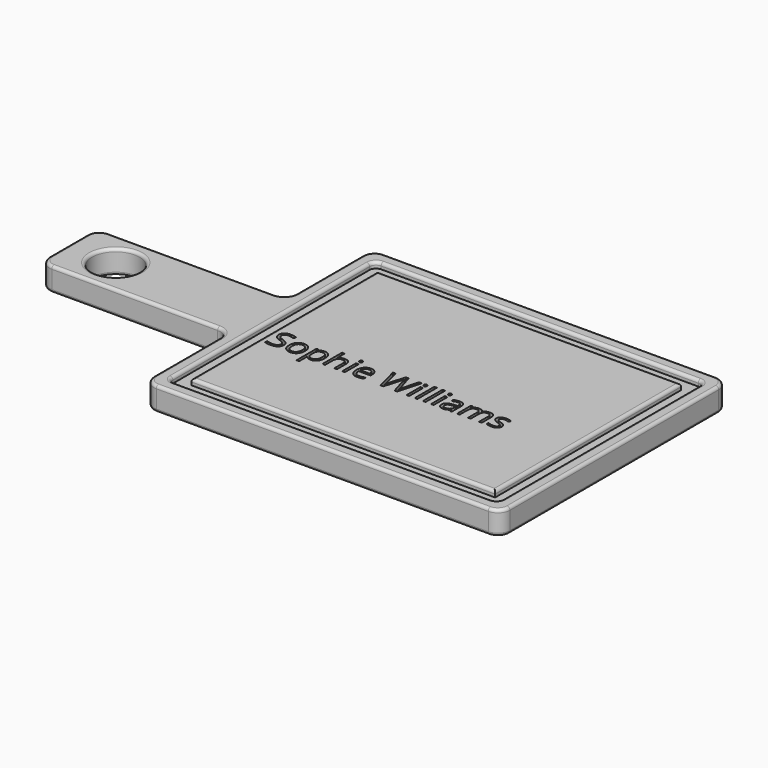
from build123d import *

# Parameters (mm, degrees)
F1_DEPTH      = 25.4
F2_R          = 25.4
F3_DEPTH      = 25.4
F5_DEPTH      = 6.35
F6_R          = 6.8679547422
F7_R          = 12.8774151417
F8_R          = 3.175
F9_TEXT_SIZE  = 41.9478889638
F10_DEPTH     = 5.08
F11_TEXT_SIZE = 34.4487062663
F12_DEPTH     = 5.08


# Not quite as in the source:
# - Text() gives the source's letters only with a copy of the font that has no kerning and outlines rounded to 1/6400 em; it was checked with that copy


with BuildPart() as f1:
    # F0 (on Top) → F1 (new body)
    with BuildSketch(Plane.XY):
        Polygon((0, 31.6785983741), (0, 0), (381, 0), (381, 304.8), (0, 304.8), (0, 190.5), (0, 152.4), (0, 114.3), align=None)
        Polygon((-203.2, 114.3), (0, 114.3), (0, 152.4), (0, 190.5), (-203.2, 190.5), align=None)
    extrude(amount=F1_DEPTH)

    # F2 (on face) → F3 (cut)
    with BuildSketch(Plane.XY.offset(25.4)):
        with Locations((-152.4, 152.4)):
            Circle(F2_R)
    extrude(amount=-F3_DEPTH, mode=Mode.SUBTRACT)

    # F4 (on face) → F5 (cut)
    with BuildSketch(Plane.XY.offset(25.4)):
        Polygon((13.9700136662, 190.5), (13.9700136662, 114.3), (13.9700136662, 13.9700136662), (367.0299863338, 13.9700136662), (367.0299863338, 290.8299863338), (13.9700136662, 290.8299863338), align=None)
        Polygon((27.940001297, 114.3), (27.940001297, 190.5), (27.940001297, 276.859998703), (353.059998703, 276.859998703), (353.059998703, 27.940001297), (27.940001297, 27.940001297), align=None, mode=Mode.SUBTRACT)
    extrude(amount=-F5_DEPTH, mode=Mode.SUBTRACT)

    # F6
    f6_edges = [f1.edges().sort_by_distance(p)[0] for p in [
        (13.970014, 290.829986, 22.225),
        (367.029986, 290.829986, 22.225),
        (367.029986, 13.970014, 22.225),
        (13.970014, 13.970014, 22.225),
    ]]
    fillet(f6_edges, radius=F6_R)

    # F7
    f7_edges = [f1.edges().sort_by_distance(p)[0] for p in [
        (381, 304.8, 12.7),
        (0, 304.8, 12.7),
        (0, 0, 12.7),
        (381, 0, 12.7),
        (-203.2, 114.3, 12.7),
        (-203.2, 190.5, 12.7),
        (0, 114.3, 12.7),
        (0, 190.5, 12.7),
    ]]
    fillet(f7_edges, radius=F7_R)

    # F8
    f8_edges = [f1.edges().sort_by_distance(p)[0] for p in [
        (190.5, 276.859999, 25.4),
        (353.059999, 152.4, 25.4),
        (190.5, 27.940001, 25.4),
        (27.940001, 152.4, 25.4),
        (190.5, 0, 25.4),
        (3.771708, 3.771708, 25.4),
        (377.228292, 3.771708, 25.4),
        (0, 57.15, 25.4),
        (381, 152.4, 25.4),
        (-3.771708, 110.528292, 25.4),
        (377.228292, 301.028292, 25.4),
        (-101.6, 114.3, 25.4),
        (190.5, 304.8, 25.4),
        (-199.428292, 118.071708, 25.4),
        (3.771708, 301.028292, 25.4),
        (-203.2, 152.4, 25.4),
        (0, 247.65, 25.4),
        (-199.428292, 186.728292, 25.4),
        (-3.771708, 194.271708, 25.4),
        (-101.6, 190.5, 25.4),
        (190.5, 13.970014, 25.4),
        (15.981591, 15.981591, 25.4),
        (365.018409, 15.981591, 25.4),
        (13.970014, 152.4, 25.4),
        (367.029986, 152.4, 25.4),
        (15.981591, 288.818409, 25.4),
        (365.018409, 288.818409, 25.4),
        (190.5, 290.829986, 25.4),
        (-177.8, 152.4, 25.4),
        (190.5, 0, 0),
        (3.771708, 3.771708, 0),
        (377.228292, 3.771708, 0),
        (0, 57.15, 0),
        (381, 152.4, 0),
        (-3.771708, 110.528292, 0),
        (377.228292, 301.028292, 0),
        (-101.6, 114.3, 0),
        (190.5, 304.8, 0),
        (-199.428292, 118.071708, 0),
        (3.771708, 301.028292, 0),
        (-203.2, 152.4, 0),
        (0, 247.65, 0),
        (-199.428292, 186.728292, 0),
        (-3.771708, 194.271708, 0),
        (-101.6, 190.5, 0),
        (-177.8, 152.4, 0),
    ]]
    fillet(f8_edges, radius=F8_R)

    # F9 (on face) → F10 (cut)
    with BuildSketch(Plane.XY.offset(25.4)):
        with Locations((31.115001297, 152.4)):
            Text('Sophie Williams', F9_TEXT_SIZE, font='Open Sans', text_align=(TextAlign.LEFT, TextAlign.BOTTOM))
    extrude(amount=F10_DEPTH, mode=Mode.SUBTRACT)

    # F11 (on face) → F12 (cut)
    with BuildSketch(Plane.XY.offset(25.4)):
        with Locations((33.3014011315, 117.0367279033)):
            Text('Sophie Williams', F11_TEXT_SIZE, font='Open Sans', text_align=(TextAlign.LEFT, TextAlign.BOTTOM))
    extrude(amount=-F12_DEPTH, mode=Mode.SUBTRACT)


solid = f1.part
